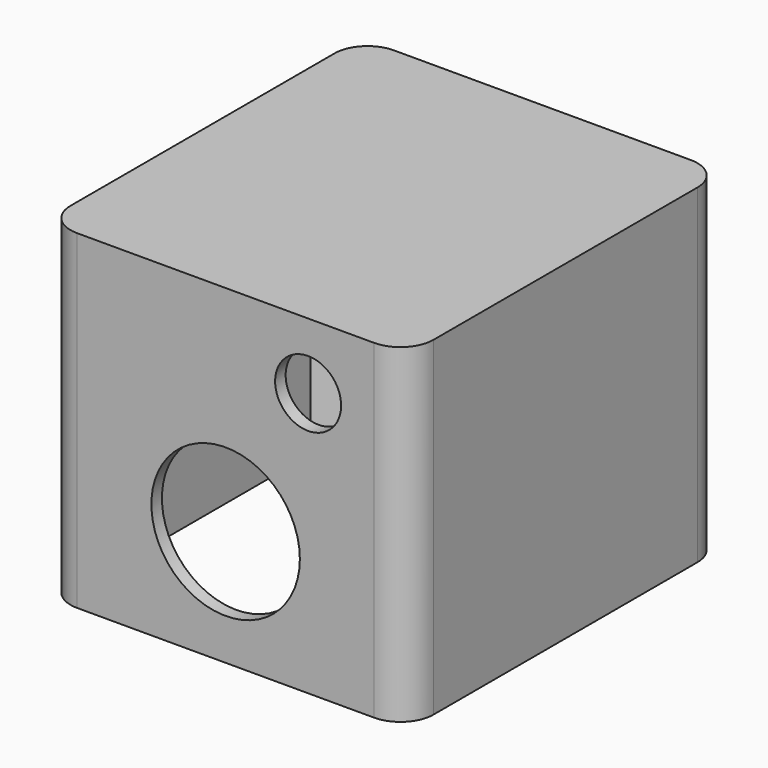
from build123d import *

# Parameters (mm, degrees)
F0_W          = 69.85
F0_H          = 63.5
F1_DEPTH      = 76.2
F2_T          = -2.54
F3_R          = 14.2875
F3_R_2        = 6.35
F4_DEPTH      = 2.54
F5_R          = 6.35
F7_DEPTH      = 38.1
F9_T1_DEPTH   = 83.2812601365
F9_2_T1_DEPTH = 83.2812601365


# Not quite as in the source:
# - a fillet or chamfer that OpenCascade refuses, or shapes differently, is made with other operations: its cross-section is extruded or revolved along the edge and cut away or added


with BuildPart() as f1:
    # F0 (on Front) → F1 (new body)
    with BuildSketch(Plane.XZ):
        with Locations((0, 9.525)):
            Rectangle(F0_W, F0_H)
    extrude(amount=-F1_DEPTH)

    # F2
    f2_openings = [f1.faces().sort_by_distance(p)[0] for p in [
        (0, 38.1, -22.225),
    ]]
    offset(amount=F2_T, openings=f2_openings)

    # F3 (on face) → F4 (cut, through all)
    with BuildSketch(Plane.XZ):
        Circle(F3_R)
        with Locations((15.875, 28.575)):
            Circle(F3_R_2)
    extrude(amount=-F4_DEPTH, mode=Mode.SUBTRACT)

    # F5
    f5_edges = [f1.edges().sort_by_distance(p)[0] for p in [
        (-34.925, 0, 9.525),
        (34.925, 0, 9.525),
        (-34.925, 76.2, 9.525),
        (34.925, 76.2, 9.525),
    ]]
    fillet(f5_edges, radius=F5_R)



with BuildPart() as f7:
    # F6 (on face) → F7 (new body)
    with BuildSketch(Plane(origin=(0, 0, -22.225), x_dir=(1, 0, 0), z_dir=(0, 0, -1))):
        Polygon((32.385, -2.54), (19.685, -2.54), (32.385, -15.24), align=None)
    extrude(amount=-F7_DEPTH)


with BuildPart() as f8_1:
    # F8: instance of F7
    add(f7.part.mirror(Plane.YZ))

    # F9: chamfer of 12.7 on 1 edges, made by hand

    # F9_s2 → F9_t1 (cut)
    with BuildSketch(Plane(origin=(11.9818718941, -11.9818718941, 0), x_dir=(0, 0, 1), z_dir=(-0.7071067812, 0.7071067812, 0))):
        Polygon((3.175, -12.1233457634), (15.875, -24.8233457634), (15.875, -12.1233457634), align=None)
    extrude(amount=F9_T1_DEPTH, mode=Mode.SUBTRACT)


with BuildPart() as f7_1:
    add(f7.part)

    # F9#2: chamfer of 12.7 on 1 edges, made by hand

    # F9_2_s2 → F9_2_t1 (cut)
    with BuildSketch(Plane(origin=(-11.9818718941, -11.9818718941, 0), x_dir=(0, 0, 1), z_dir=(0.7071067812, 0.7071067812, 0))):
        Polygon((3.175, 12.1233457634), (15.875, 24.8233457634), (15.875, 12.1233457634), align=None)
    extrude(amount=F9_2_T1_DEPTH, mode=Mode.SUBTRACT)


with BuildPart() as f1_1:
    add(f1.part)

    add(f7_1.part)  # F11 merges F7

    add(f8_1.part)  # F11 merges F8_1
    # F11: F8_1, F7 across plane
    add(f8_1.part.mirror(Plane(origin=(0, 38.1, 9.525), x_dir=(1, 0, 0), z_dir=(0, 1, 0))))
    add(f7_1.part.mirror(Plane(origin=(0, 38.1, 9.525), x_dir=(1, 0, 0), z_dir=(0, 1, 0))))


solid = f1_1.part
